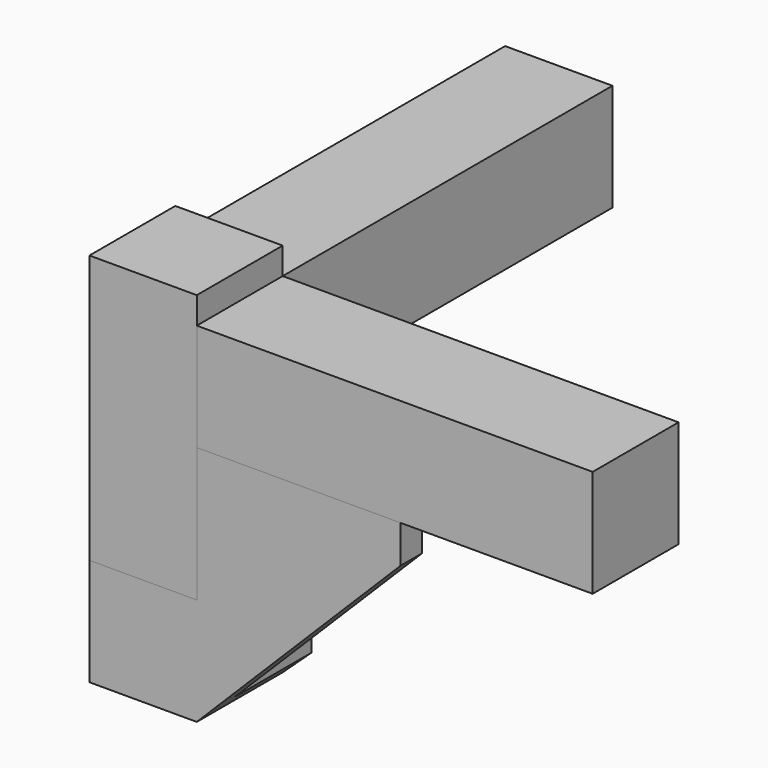
from build123d import *

# Parameters (mm, degrees)
F0_W          = 20
F0_H          = 76.8000064468
F1_DEPTH      = 20
F0_W_2        = 73.7599998636
F0_H_2        = 20
F2_DEPTH      = 25
F2_DEPTH_BACK = 25
F3_W          = 20
F3_H          = 20
F4_DEPTH      = 20
F5_DEPTH      = 5
F7_DEPTH      = 5
F9_DEPTH      = 45
F10_DEPTH     = 25
F11_DEPTH     = 25
F12_DEPTH     = 25


with BuildPart() as f1:
    # F0 (on Top) → F1 (new body)
    with BuildSketch(Plane.XY):
        with Locations((-10, 38.4000032234)):
            Rectangle(F0_W, F0_H)
    extrude(amount=F1_DEPTH)


with BuildPart() as f1b:
    # F0 (on Top) → F1, piece 2 (new body)
    with BuildSketch(Plane.XY):
        with Locations((36.8799999318, -10)):
            Rectangle(F0_W_2, F0_H_2)
    extrude(amount=F1_DEPTH)


with BuildPart() as f2:
    # F0 (on Top) → F2 (new body, two sides)
    with BuildSketch(Plane.XY) as f2_sk:
        with Locations((-10, -10)):
            Rectangle(F0_W, F0_H_2)
    extrude(amount=-F2_DEPTH)
    extrude(f2_sk.sketch, amount=F2_DEPTH_BACK)


with BuildPart() as f4:
    # F3 (on face) → F4 (new body)
    with BuildSketch(Plane(origin=(-20, 0, 0), x_dir=(0, -1, 0), z_dir=(-1, 0, 0))):
        with Locations((10, -35)):
            Rectangle(F3_W, F3_H)
    extrude(amount=-F4_DEPTH)

    # F3 (on face) → F5 (join)
    with BuildSketch(Plane(origin=(-20, 0, 0), x_dir=(0, -1, 0), z_dir=(-1, 0, 0))):
        Polygon((0, -45), (0, -25), (0, 0), (-38, 0), (-38, -7), align=None)
    extrude(amount=-F5_DEPTH)

    # F6 (on face) → F7 (join)
    with BuildSketch(Plane.XZ.offset(20)):
        Polygon((0, -25), (0, -45), (38, -7), (38, 0), (0, 0), align=None)
    extrude(amount=-F7_DEPTH)

    # F8 (on Top) → F9 (join)
    with BuildSketch(Plane.XY):
        Polygon((3, 3), (-15, 3), (-15, 0), (0, 0), (0, -15), (3, -15), align=None)
    extrude(amount=-F9_DEPTH)

    # F10 (cut): a face of the model
    f10_faces = [f4.faces().sort_by_distance(p)[0] for p in [
        (-15, 2, -44),
    ]]
    extrude(f10_faces, amount=-F10_DEPTH, mode=Mode.SUBTRACT)

    # F11 (cut): a face of the model
    f11_faces = [f4.faces().sort_by_distance(p)[0] for p in [
        (2, -15, -44),
    ]]
    extrude(f11_faces, amount=-F11_DEPTH, mode=Mode.SUBTRACT)

    # F12 (cut): a face of the model
    f12_faces = [f4.faces().sort_by_distance(p)[0] for p in [
        (-15, 16.3333333333, -14.3333333333),
    ]]
    extrude(f12_faces, amount=-F12_DEPTH, mode=Mode.SUBTRACT)


solid = Compound([f1.part, f1b.part, f2.part, f4.part])
